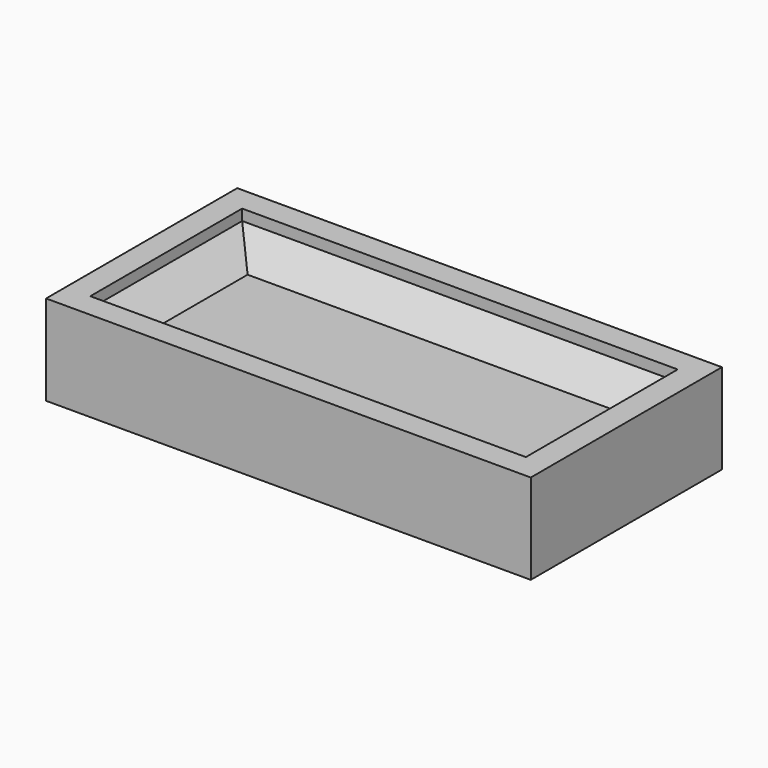
from build123d import *

# Parameters (mm, degrees)
F0_W         = 31.9
F0_H         = 13.9
F1_DEPTH     = 0.5
F0_W_2       = 35.5
F0_H_2       = 17.5
F2_DEPTH     = 3.3
F3_SIZE      = 2
F4_TEXT_SIZE = 7.0899986706
F5_DEPTH     = 0.5


# Not quite as in the source:
# - Text() gives the source's letters only with a copy of the font that has no kerning and outlines rounded to 1/6400 em; it was checked with that copy


with BuildPart() as f1:
    # F0 (on Top) → F1 (new body, symmetric)
    with BuildSketch(Plane.XY):
        Rectangle(F0_W, F0_H)
    extrude(amount=F1_DEPTH, both=True)

    # F0 (on Top) → F2 (join, symmetric)
    with BuildSketch(Plane.XY):
        Rectangle(F0_W_2, F0_H_2)
        Rectangle(F0_W, F0_H, mode=Mode.SUBTRACT)
    extrude(amount=F2_DEPTH, both=True)

    # F3
    f3_edges = [f1.edges().sort_by_distance(p)[0] for p in [
        (0, 6.95, 0.5),
        (15.95, 0, 0.5),
        (0, -6.95, 0.5),
        (-15.95, 0, 0.5),
        (0, -6.95, -0.5),
        (-15.95, 0, -0.5),
        (0, 6.95, -0.5),
        (15.95, 0, -0.5),
    ]]
    chamfer(f3_edges, length=F3_SIZE)

    # F4 (on face) → F5 (join)
    with BuildSketch(Plane(origin=(0, 0, -0.5), x_dir=(1, 0, 0), z_dir=(0, 0, -1))):
        with Locations((-12.5, -2.5547990429)):
            Text('MIKKEL', F4_TEXT_SIZE, font='Open Sans', text_align=(TextAlign.LEFT, TextAlign.BOTTOM))
    extrude(amount=F5_DEPTH)


solid = f1.part
